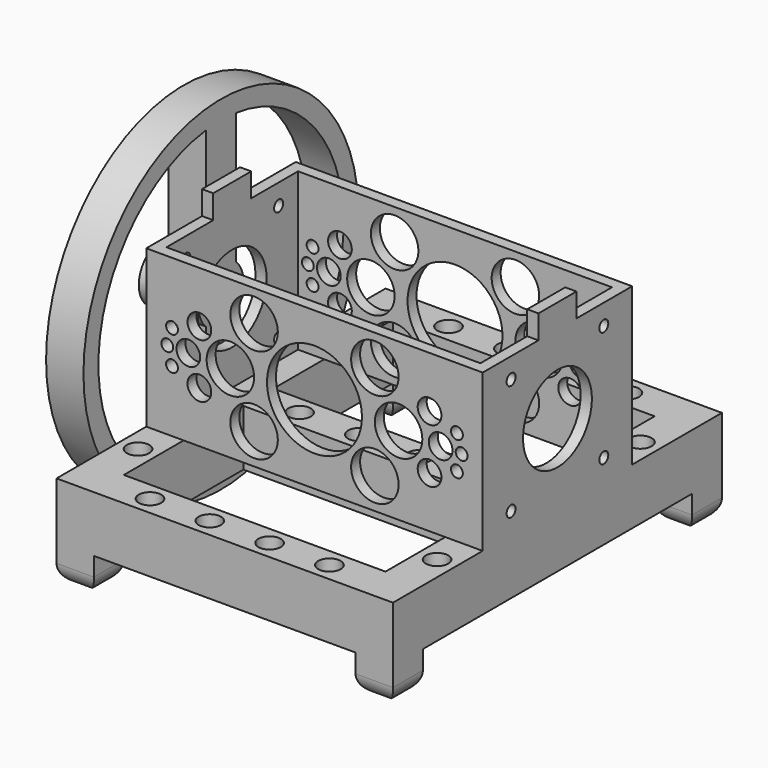
from build123d import *

# Parameters (mm, degrees)
F0_W      = 90
F0_H      = 110
F0_W_2    = 70
F0_H_2    = 40
F1_DEPTH  = 15
F2_W      = 3
F2_H      = 3
F2_W_2    = 7
F2_H_2    = 44
F2_W_3    = 70
F3_DEPTH  = 42
F4_W      = 10
F4_H      = 10
F5_DEPTH  = 10
F6_R      = 11.5
F6_R_2    = 1.5
F7_DEPTH  = 90
F8_R      = 4.99999
F9_R      = 12.7
F9_R_2    = 6.35
F9_R_3    = 3.175
F9_R_4    = 1.5875
F10_DEPTH = 80.001
F11_W     = 3
F11_H     = 12.7
F12_DEPTH = 6.35
F13_R     = 46
F14_DEPTH = 10
F15_R     = 7.5
F15_W     = 5.5
F15_H     = 2.4
F16_DEPTH = 6
F18_R     = 1.5
F19_DEPTH = 12.8
F20_W     = 5.5
F20_H     = 2.4
F21_DEPTH = 2.5
F22_R     = 3
F23_DEPTH = 25.4


# Not quite as in the source:
# - a fillet or chamfer is up to 0.001 mm smaller than in the source, because OpenCascade refuses the exact size


with BuildPart() as f1:
    # F0 (on Top) → F1 (new body)
    with BuildSketch(Plane.XY):
        Rectangle(F0_W, F0_H)
        with Locations((0, -25)):
            Rectangle(F0_W_2, F0_H_2, mode=Mode.SUBTRACT)
        with Locations((0, 25)):
            Rectangle(F0_W_2, F0_H_2, mode=Mode.SUBTRACT)
    extrude(amount=F1_DEPTH)

    # F2 (on face) → F3 (join)
    with BuildSketch(Plane.XY.offset(15)):
        with Locations((43.5, 23.5)):
            Rectangle(F2_W, F2_H)
        with Locations((38.5, 23.5)):
            Rectangle(F2_W_2, F2_H)
        with Locations((43.5, 0)):
            Rectangle(F2_W, F2_H_2)
        with Locations((0, 23.5)):
            Rectangle(F2_W_3, F2_H)
        with Locations((43.5, -23.5)):
            Rectangle(F2_W, F2_H)
        with Locations((38.5, -23.5)):
            Rectangle(F2_W_2, F2_H)
        with Locations((-38.5, 23.5)):
            Rectangle(F2_W_2, F2_H)
        with Locations((0, -23.5)):
            Rectangle(F2_W_3, F2_H)
        with Locations((-43.5, 23.5)):
            Rectangle(F2_W, F2_H)
        with Locations((-38.5, -23.5)):
            Rectangle(F2_W_2, F2_H)
        with Locations((-43.5, 0)):
            Rectangle(F2_W, F2_H_2)
        with Locations((-43.5, -23.5)):
            Rectangle(F2_W, F2_H)
    extrude(amount=F3_DEPTH)

    # F4 (on face) → F5 (join)
    with BuildSketch(Plane(origin=(0, 0, 0), x_dir=(1, 0, 0), z_dir=(0, 0, -1))):
        with Locations((-40, -50)):
            Rectangle(F4_W, F4_H)
        with Locations((-40, 50)):
            Rectangle(F4_W, F4_H)
        with Locations((40, 50)):
            Rectangle(F4_W, F4_H)
        with Locations((40, -50)):
            Rectangle(F4_W, F4_H)
    extrude(amount=F5_DEPTH)

    # F6 (on face) → F7 (cut, through all)
    with BuildSketch(Plane(origin=(-45, 0, 0), x_dir=(0, -1, 0), z_dir=(-1, 0, 0))):
        with Locations((0, 36)):
            Circle(F6_R)
        with Locations((-15.5, 20.5)):
            Circle(F6_R_2)
        with Locations((15.5, 20.5)):
            Circle(F6_R_2)
        with Locations((15.5, 51.5)):
            Circle(F6_R_2)
        with Locations((-15.5, 51.5)):
            Circle(F6_R_2)
    extrude(amount=-F7_DEPTH, mode=Mode.SUBTRACT)

    # F8 (radius 5 in the source; OpenCascade refuses exactly that, so slightly less here)
    f8_edges = [f1.edges().sort_by_distance(p)[0] for p in [
        (35, -50, -10),
        (40, -45, -10),
        (45, -50, -10),
        (40, -55, -10),
        (-45, -50, -10),
        (-40, -45, -10),
        (-35, -50, -10),
        (-40, -55, -10),
        (45, 50, -10),
        (40, 45, -10),
        (35, 50, -10),
        (40, 55, -10),
        (-35, 50, -10),
        (-40, 45, -10),
        (-45, 50, -10),
        (-40, 55, -10),
    ]]
    fillet(f8_edges, radius=F8_R)

    # F9 (on face) → F10 (cut, through all)
    with BuildSketch(Plane.XZ.offset(25)):
        with Locations((0, 36)):
            Circle(F9_R)
        with Locations((22.5, 36)):
            Circle(F9_R_2)
        with Locations((-22.5, 36)):
            Circle(F9_R_2)
        with Locations((33.75, 36)):
            Circle(F9_R_3)
        with Locations((-33.75, 36)):
            Circle(F9_R_3)
        with Locations((16.153611, 23.297113)):
            Circle(F9_R_2)
        with Locations((16.153611, 48.702887)):
            Circle(F9_R_2)
        with Locations((-16.153611, 48.702887)):
            Circle(F9_R_2)
        with Locations((-16.153611, 23.297113)):
            Circle(F9_R_2)
        with Locations((30.788472, 28.730072)):
            Circle(F9_R_3)
        with Locations((30.788472, 43.269928)):
            Circle(F9_R_3)
        with Locations((-30.788472, 43.269928)):
            Circle(F9_R_3)
        with Locations((-30.788472, 28.730072)):
            Circle(F9_R_3)
        with Locations((39.375, 36)):
            Circle(F9_R_4)
        with Locations((38.105903, 31.500554)):
            Circle(F9_R_4)
        with Locations((38.105903, 40.499446)):
            Circle(F9_R_4)
        with Locations((-38.105903, 40.499446)):
            Circle(F9_R_4)
        with Locations((-38.105903, 31.500554)):
            Circle(F9_R_4)
        with Locations((-39.375, 36)):
            Circle(F9_R_4)
    extrude(amount=-F10_DEPTH, mode=Mode.SUBTRACT)

    # F11 (on face) → F12 (join)
    with BuildSketch(Plane.XY.offset(57)):
        with Locations((43.5, 0)):
            Rectangle(F11_W, F11_H)
        with Locations((-43.5, 0)):
            Rectangle(F11_W, F11_H)
    extrude(amount=F12_DEPTH)

    # F20 (on face) → F21 (cut)
    with BuildSketch(Plane(origin=(-61, 0, 0), x_dir=(0, -1, 0), z_dir=(-1, 0, 0))):
        with Locations((0, 40.2)):
            Rectangle(F20_W, F20_H)
    extrude(amount=-F21_DEPTH, mode=Mode.SUBTRACT)

    # F22 (on face) → F23 (cut)
    with BuildSketch(Plane.XY.offset(15)):
        with Locations((-24, -50)):
            Circle(F22_R)
        with Locations((-8, -50)):
            Circle(F22_R)
        with Locations((8, -50)):
            Circle(F22_R)
        with Locations((24, -50)):
            Circle(F22_R)
        with Locations((24, 49.822)):
            Circle(F22_R)
        with Locations((8, 49.822)):
            Circle(F22_R)
        with Locations((-8, 49.822)):
            Circle(F22_R)
        with Locations((-24, 49.822)):
            Circle(F22_R)
        with Locations((-8, 0)):
            Circle(F22_R)
        with Locations((-24, 0)):
            Circle(F22_R)
        with Locations((8, 0)):
            Circle(F22_R)
        with Locations((24, 0)):
            Circle(F22_R)
        with Locations((40, -34)):
            Circle(F22_R)
        with Locations((40, 34)):
            Circle(F22_R)
        with Locations((-40, 34)):
            Circle(F22_R)
        with Locations((-40, -34)):
            Circle(F22_R)
    extrude(amount=-F23_DEPTH, mode=Mode.SUBTRACT)


with BuildPart() as f14:
    # F13 (on face) → F14 (new body)
    with BuildSketch(Plane(origin=(-45, 0, 0), x_dir=(0, -1, 0), z_dir=(-1, 0, 0))):
        with Locations((0, 36)):
            Circle(F13_R)
        with BuildLine():
            ThreePointArc((1.5, 38), (0, 33.5), (-1.5, 38))
            Line((-1.5, 38), (1.5, 38))
        make_face(mode=Mode.SUBTRACT)
        with BuildLine():
            ThreePointArc((-5, -4.69398), (-41, 36), (-5, 76.69398))
            Line((-5, 76.69398), (-5, 41.59017))
            ThreePointArc((-5, 41.59017), (-7.5, 36), (-5, 30.40983))
            Line((-5, 30.40983), (-5, -4.69398))
        make_face(mode=Mode.SUBTRACT)
        with BuildLine():
            Line((5, 41.59017), (5, 76.69398))
            ThreePointArc((5, 76.69398), (41, 36), (5, -4.69398))
            Line((5, -4.69398), (5, 30.40983))
            ThreePointArc((5, 30.40983), (7.5, 36), (5, 41.59017))
        make_face(mode=Mode.SUBTRACT)
    extrude(amount=F14_DEPTH)

    # F15 (on face) → F16 (join)
    with BuildSketch(Plane(origin=(-55, 0, 0), x_dir=(0, -1, 0), z_dir=(-1, 0, 0))):
        with Locations((0, 36)):
            Circle(F15_R)
        with BuildLine():
            ThreePointArc((1.5, 38), (0, 33.5), (-1.5, 38))
            Line((-1.5, 38), (1.5, 38))
        make_face(mode=Mode.SUBTRACT)
        with Locations((0, 40.2)):
            Rectangle(F15_W, F15_H, mode=Mode.SUBTRACT)
    extrude(amount=F16_DEPTH)

    # F18 (on offset) → F19 (cut, through all)
    with BuildSketch(Plane.XY.offset(50.8)):
        with Locations((-58, 0)):
            Circle(F18_R)
    extrude(amount=-F19_DEPTH, mode=Mode.SUBTRACT)


solid = Compound([f1.part, f14.part])
